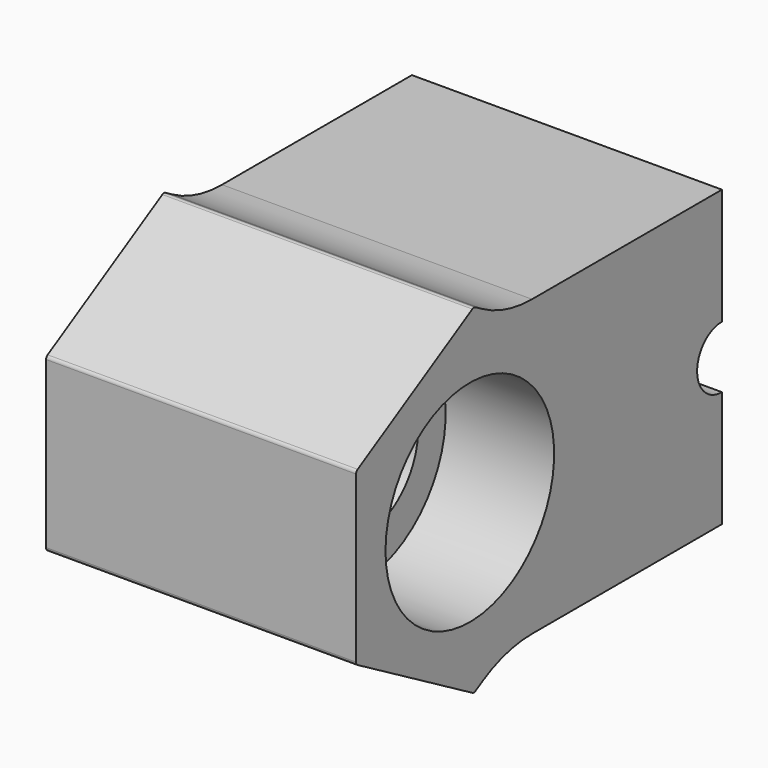
from build123d import *

# Parameters (mm, degrees)
F1_DEPTH  = 20
F4_R      = 4.25
F5_DEPTH  = 20.001
F6_R      = 6.8
F6_R_2    = 4.25
F7_DEPTH  = 7
F10_R     = 8
F12_DEPTH = 20.001
F13_R     = 0.25


# Not quite as in the source:
# - a feature names something its author has since deleted; it is built from what else it names


with BuildPart() as f1:
    # F0 (on Right) → F1 (new body)
    with BuildSketch(Plane.YZ):
        Polygon((2.5455173281, 9.5), (0, 10.9696551146), (-9.5, 5.4848275573), (-9.5, -5.4848275573), (0, -10.9696551146), (2.5455173281, -9.5), (9.5, -5.4848275573), (9.5, 0), (9.5, 5.4848275573), align=None)
        Polygon((20, 9.5), (2.5455173281, 9.5), (9.5, 5.4848275573), (9.5, 0), (20, 0), align=None)
        Polygon((20, 0), (9.5, 0), (9.5, -5.4848275573), (2.5455173281, -9.5), (20, -9.5), align=None)
    extrude(amount=F1_DEPTH)

    # F4 (on face) → F5 (cut, through all)
    with BuildSketch(Plane(origin=(0, 0, 0), x_dir=(0, -1, 0), z_dir=(-1, 0, 0))):
        Circle(F4_R)
    extrude(amount=-F5_DEPTH, mode=Mode.SUBTRACT)


with BuildPart() as f7:
    # F6 (on face) → F7 (new body)
    with BuildSketch(Plane(origin=(0, 0, 0), x_dir=(0, -1, 0), z_dir=(-1, 0, 0))):
        with Locations((0.3292050309, 0)):
            Circle(F6_R)
        Circle(F6_R_2, mode=Mode.SUBTRACT)
        Circle(F6_R_2)
    extrude(amount=-F7_DEPTH)


with BuildPart() as f8_1:
    # F8: instance of F7
    add(f7.part.mirror(Plane(origin=(10, 5.820047307, 0), x_dir=(0, 1, 0), z_dir=(1, 0, 0))))


with BuildPart() as f1_1:
    add(f1.part)

    # F9: cut F7, F8_1
    add(f7.part, mode=Mode.SUBTRACT)
    add(f8_1.part, mode=Mode.SUBTRACT)

    # F10
    f10_edges = [f1_1.edges().sort_by_distance(p)[0] for p in [
        (10, 2.545517, -9.5),
        (10, 2.545517, 9.5),
    ]]
    fillet(f10_edges, radius=F10_R)

    # F11 (on face) → F12 (cut, through all)
    with BuildSketch(Plane.YZ.offset(20)):
        with BuildLine():
            Line((20, 0), (20, 2))
            ThreePointArc((20, 2), (18.5857864376, 1.4142135624), (18, 0))
            Line((18, 0), (20, 0))
        make_face()
        with BuildLine():
            ThreePointArc((18, 0), (18.5857864376, -1.4142135624), (20, -2))
            Line((20, -2), (20, 0))
            Line((20, 0), (18, 0))
        make_face()
        with BuildLine():
            ThreePointArc((20, -2), (21.4142135624, -1.4142135624), (22, 0))
            ThreePointArc((22, 0), (21.4142135624, 1.4142135624), (20, 2))
            Line((20, 2), (20, 0))
            Line((20, 0), (20, -2))
        make_face()
    extrude(amount=-F12_DEPTH, mode=Mode.SUBTRACT)

    # F13
    f13_edges = [f1_1.edges().sort_by_distance(p)[0] for p in [
        (10, -9.5, -5.484828),
        (10, -9.5, 5.484828),
        (10, 0, 10.969655),
        (10, 0, -10.969655),
    ]]
    fillet(f13_edges, radius=F13_R)


solid = f1_1.part
